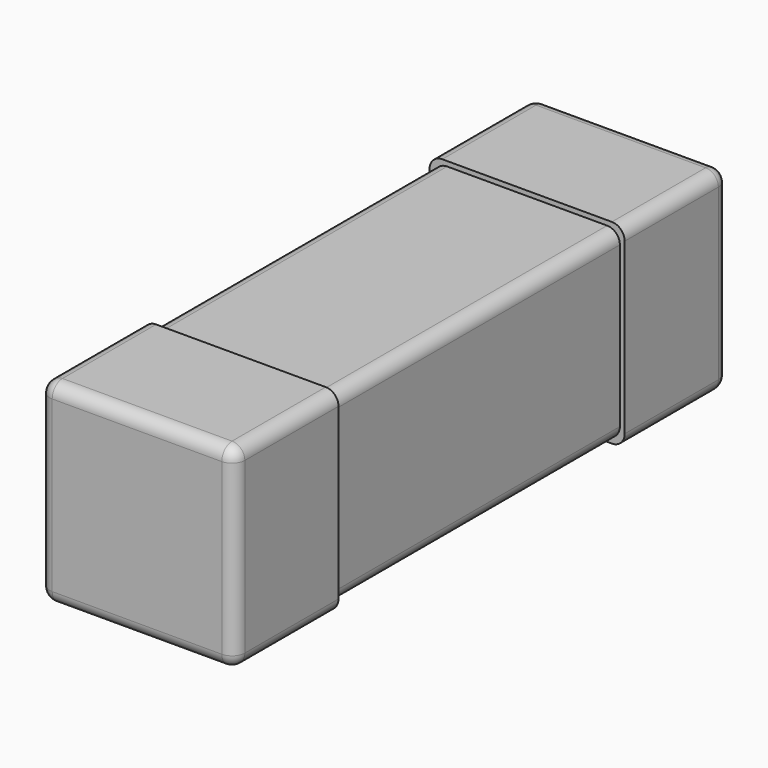
from build123d import *

# Parameters (mm, degrees)
F2_W     = 2.9
F2_H     = 2.9
F3_DEPTH = 2.795
F4_W     = 3.05
F4_H     = 3.05
F5_DEPTH = 2.03
F6_R     = 0.2
F6_2_R   = 0.2
F6_3_R   = 0.2


# Not quite as in the source:
# - two fillets or chamfers of one size are made in one step
# - a pattern or mirror of a feature is missing from the dataset's text; its kind, count and spacing are read off the source's solid


with BuildPart() as f3:
    # F2 (on Front) → F3 (new body, symmetric)
    with BuildSketch(Plane.XZ):
        Rectangle(F2_W, F2_H)
    extrude(amount=F3_DEPTH, both=True)

    # F6#2
    f6_2_edges = [f3.edges().sort_by_distance(p)[0] for p in [
        (1.45, 0, 1.45),
        (1.45, 0, -1.45),
        (-1.45, 0, -1.45),
        (-1.45, 0, 1.45),
    ]]
    fillet(f6_2_edges, radius=F6_2_R)


with BuildPart() as f5:
    # F4 (on face) → F5 (new body)
    with BuildSketch(Plane.XZ.offset(2.795)):
        Rectangle(F4_W, F4_H)
    extrude(amount=F5_DEPTH)


with BuildPart() as f5_copies_1:
    # F5_copies: instance of F5
    add(f5.part.mirror(Plane.ZX))

    # F6#3
    f6_3_edges = [f5_copies_1.edges().sort_by_distance(p)[0] for p in [
        (1.525, 3.81, -1.525),
        (1.525, 3.81, 1.525),
        (1.525, 4.825, 0),
        (-1.525, 3.81, 1.525),
        (0, 4.825, 1.525),
        (-1.525, 3.81, -1.525),
        (-1.525, 4.825, 0),
        (0, 4.825, -1.525),
    ]]
    fillet(f6_3_edges, radius=F6_3_R)


with BuildPart() as f5_1:
    add(f5.part)

    # F6
    f6_edges = [f5_1.edges().sort_by_distance(p)[0] for p in [
        (1.525, -4.825, 0),
        (0, -4.825, 1.525),
        (-1.525, -4.825, 0),
        (0, -4.825, -1.525),
        (1.525, -3.81, -1.525),
        (-1.525, -3.81, -1.525),
        (1.525, -3.81, 1.525),
        (-1.525, -3.81, 1.525),
    ]]
    fillet(f6_edges, radius=F6_R)


solid = Compound([f3.part, f5_copies_1.part, f5_1.part])
